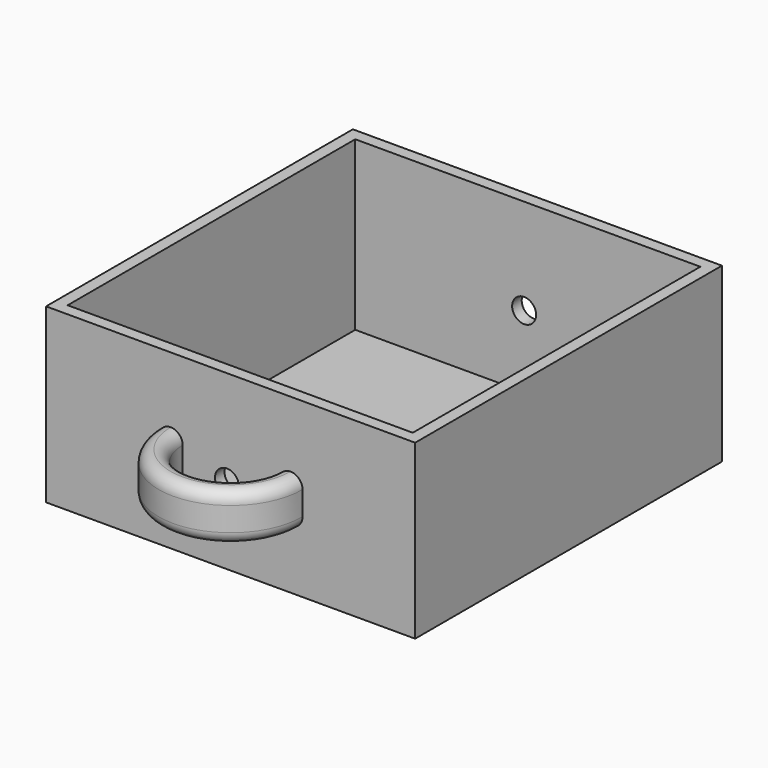
from build123d import *

# Parameters (mm, degrees)
F0_W      = 97.79
F0_H      = 45.72
F1_DEPTH  = 101.6
F2_W      = 91.44
F2_H      = 95.25
F3_DEPTH  = 44.45
F4_W      = 19.05
F4_H      = 6.35
F5_ANGLE  = 180
F7_DEPTH  = 25.4
F8_R      = 3.17499
F10_D     = 6.35
F10_DEPTH = 101.601


# Not quite as in the source:
# - a fillet or chamfer is up to 0.001 mm smaller than in the source, because OpenCascade refuses the exact size


with BuildPart() as f1:
    # F0 (on Front) → F1 (new body)
    with BuildSketch(Plane.XZ):
        with Locations((15.4838143581, 4.6649015626)):
            Rectangle(F0_W, F0_H)
    extrude(amount=-F1_DEPTH)

    # F2 (on face) → F3 (cut)
    with BuildSketch(Plane.XY.offset(27.5249015626)):
        with Locations((15.4838143581, 50.8)):
            Rectangle(F2_W, F2_H)
    extrude(amount=-F3_DEPTH, mode=Mode.SUBTRACT)

    # F4 (on face) → F5 (revolve)
    with BuildSketch(Plane.XZ):
        with Locations((5.9588143581, 6.8874015626)):
            Rectangle(F4_W, F4_H)
        with Locations((5.9588143581, 0.5374015626)):
            Rectangle(F4_W, F4_H)
    revolve(axis=Axis((15.4838143581, 0, 3.7124015626), (0, 0, 1)), revolution_arc=F5_ANGLE)

    # F6 (on face) → F7 (cut)
    with BuildSketch(Plane.XY.offset(10.0624015626)):
        with BuildLine():
            Line((28.1838143581, 0), (2.7838143581, 0))
            ThreePointArc((2.7838143581, 0), (15.4838143581, -12.7), (28.1838143581, 0))
        make_face()
    extrude(amount=-F7_DEPTH, mode=Mode.SUBTRACT)

    # F8 (radius 3.175 in the source; OpenCascade refuses exactly that, so slightly less here)
    f8_edges = [f1.edges().sort_by_distance(p)[0] for p in [
        (15.483814, -19.05, 10.062402),
        (15.483814, -12.7, 10.062402),
        (15.483814, -19.05, -2.637598),
        (15.483814, -12.7, -2.637598),
    ]]
    fillet(f8_edges, radius=F8_R)

    # F10 (through all, one way)
    with BuildSketch(Plane.XZ):
        with Locations((14.5096713677, 2.1249015626)):
            Circle(F10_D / 2)
    extrude(amount=-F10_DEPTH, mode=Mode.SUBTRACT)


solid = f1.part
